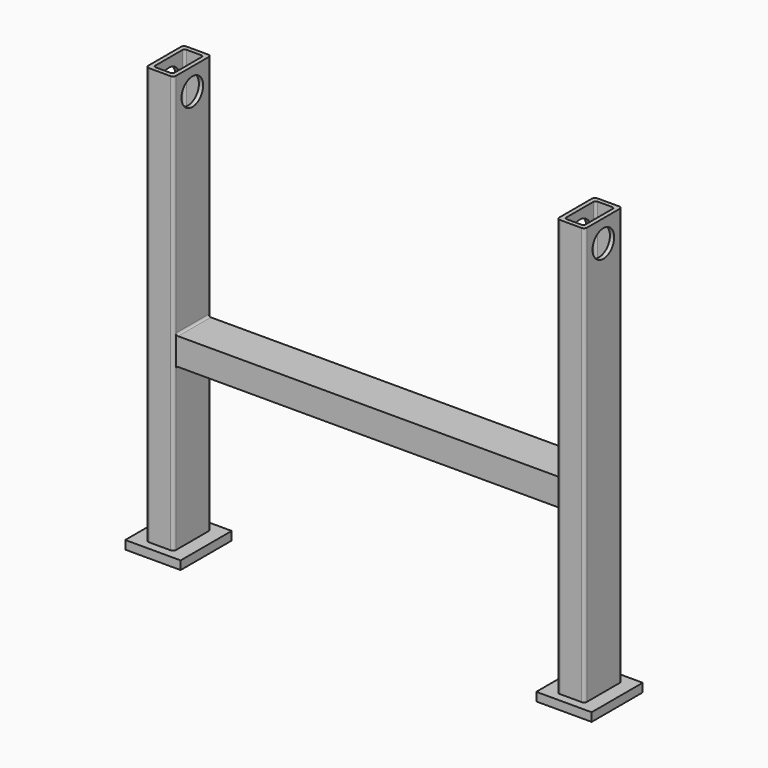
from build123d import *

# Parameters (mm, degrees)
F0_W        = 130
F0_H        = 150
F1_DEPTH    = 20
F2_W        = 65
F2_H        = 110
F2_W_2      = 45
F2_H_2      = 90
F3_DEPTH    = 980
F4_R        = 7
F5_R        = 5.08
F6_W        = 96
F6_H        = 63.5
F6_W_2      = 73.66
F6_H_2      = 45.72
F7_DEPTH    = 450
F8_T1_DEPTH = 96
F9_T1_DEPTH = 96
F13_D       = 63.5


# Not quite as in the source:
# - a fillet or chamfer that OpenCascade refuses, or shapes differently, is made with other operations: its cross-section is extruded or revolved along the edge and cut away or added


with BuildPart() as f1:
    # F0 (on Top) → F1 (new body)
    with BuildSketch(Plane.XY):
        with Locations((515, 0)):
            Rectangle(F0_W, F0_H)
    extrude(amount=F1_DEPTH)

    # F2 (on face) → F3 (join)
    with BuildSketch(Plane.XY.offset(20)):
        with Locations((515, 0)):
            Rectangle(F2_W, F2_H)
        with Locations((515, 0)):
            Rectangle(F2_W_2, F2_H_2, mode=Mode.SUBTRACT)
    extrude(amount=F3_DEPTH)

    # F4
    f4_edges = [f1.edges().sort_by_distance(p)[0] for p in [
        (547.5, -55, 510),
        (482.5, -55, 510),
        (547.5, 55, 510),
        (482.5, 55, 510),
    ]]
    fillet(f4_edges, radius=F4_R)

    # F5
    f5_edges = [f1.edges().sort_by_distance(p)[0] for p in [
        (492.5, 45, 510),
        (492.5, -45, 510),
        (537.5, -45, 510),
        (537.5, 45, 510),
    ]]
    fillet(f5_edges, radius=F5_R)

    # F6 (on face) → F7 (join)
    with BuildSketch(Plane(origin=(482.5, 0, 0), x_dir=(0, -1, 0), z_dir=(-1, 0, 0))):
        with Locations((0, 431.75)):
            Rectangle(F6_W, F6_H)
        with Locations((0.26, 431.75)):
            Rectangle(F6_W_2, F6_H_2, mode=Mode.SUBTRACT)
    extrude(amount=F7_DEPTH)

    # F8: fillet of radius 5 on 1 edges, made by hand

    # F8_s2 → F8_t1 (join)
    with BuildSketch(Plane.XZ.offset(-48)):
        with BuildLine():
            ThreePointArc((482.5, 468.5), (481.0355339059, 464.9644660941), (477.5, 463.5))
            Line((477.5, 463.5), (482.5, 463.5))
            Line((482.5, 463.5), (482.5, 468.5))
        make_face()
    extrude(amount=F8_T1_DEPTH)

    # F9: fillet of radius 5 on 1 edges, made by hand

    # F9_s2 → F9_t1 (join)
    with BuildSketch(Plane.XZ.offset(-48)):
        with BuildLine():
            ThreePointArc((482.5, 395), (481.0355339059, 398.5355339059), (477.5, 400))
            Line((477.5, 400), (482.5, 400))
            Line((482.5, 400), (482.5, 395))
        make_face()
    extrude(amount=F9_T1_DEPTH)

    # F11: F1 across face


with BuildPart() as f1_1:
    add(f1.part)
    add(f1.part.mirror(Plane(origin=(32.5, 0, 0), x_dir=(0, -1, 0), z_dir=(-1, 0, 0))))

    # F13 (through all)
    with Locations(Plane.YZ.offset(547.5)):
        with Locations((0, 947.7953910828)):
            Hole(F13_D / 2)


solid = f1_1.part
